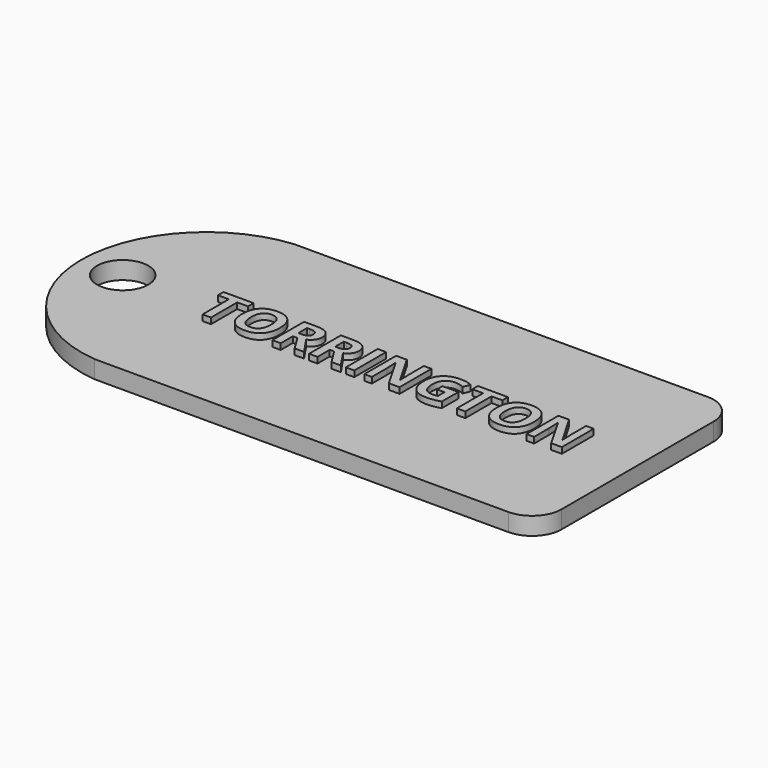
from build123d import *

# Parameters (mm, degrees)
F0_R         = 4.3404715655
F1_DEPTH     = 3
F2_TEXT_SIZE = 9.4317468918
F3_DEPTH     = 4


# Not quite as in the source:
# - Text() gives the source's letters only with a copy of the font that has no kerning and outlines rounded to 1/6400 em; it was checked with that copy


with BuildPart() as f1:
    # F0 (on Top) → F1 (new body)
    with BuildSketch(Plane.XY):
        with BuildLine():
            ThreePointArc((37.5088900328, 16.0870876908), (36.0444239387, 19.6226215968), (32.5088900328, 21.0870876908))
            Line((32.5088900328, 21.0870876908), (-37.5088900328, 21.0870876908))
            Line((-37.5088900328, 21.0870876908), (-37.5088900328, -21.0870876908))
            Line((-37.5088900328, -21.0870876908), (32.5088900328, -21.0870876908))
            ThreePointArc((32.5088900328, -21.0870876908), (36.0444239387, -19.6226215968), (37.5088900328, -16.0870876908))
            Line((37.5088900328, -16.0870876908), (37.5088900328, 16.0870876908))
        make_face()
        with BuildLine():
            Line((-37.5088900328, -21.0870876908), (-37.5088900328, 21.0870876908))
            ThreePointArc((-37.5088900328, 21.0870876908), (-56.6668901903, 0), (-37.5088900328, -21.0870876908))
        make_face()
        with Locations((-49.6386289597, 0)):
            Circle(F0_R, mode=Mode.SUBTRACT)
    extrude(amount=F1_DEPTH)

    # F2 (on Top) → F3 (join)
    with BuildSketch(Plane.XY):
        with Locations((-35.2064799517, -3.6755966721)):
            Text('TORRINGTON', F2_TEXT_SIZE, font='Open Sans', font_style=FontStyle.BOLD, text_align=(TextAlign.LEFT, TextAlign.BOTTOM))
    extrude(amount=F3_DEPTH)


solid = f1.part
